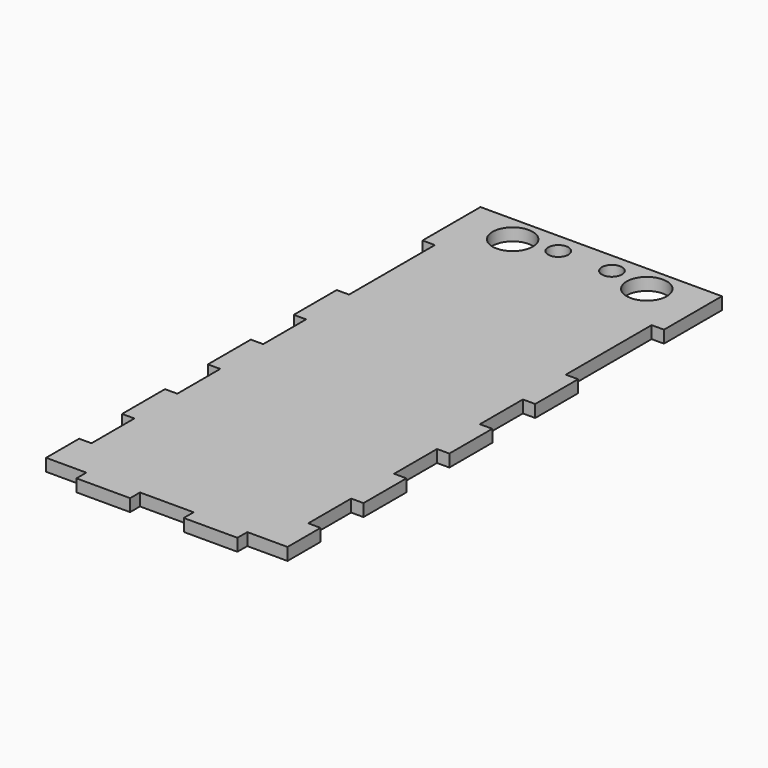
from build123d import *

# Parameters (mm, degrees)
F0_W     = 114.3
F0_H     = 262.89
F1_DEPTH = 5.842
F2_W     = 25.4
F2_H     = 5.842
F2_W_2   = 19.05
F2_W_3   = 5.842
F2_H_2   = 25.4
F3_DEPTH = 5.842
F4_R     = 4.7625
F4_R_2   = 9.525
F5_DEPTH = 5.842


# Not quite as in the source:
# - a feature names something its author has since deleted; it is built from what else it names


with BuildPart() as f1:
    # F0 (on Top) → F1 (new body)
    with BuildSketch(Plane.XY):
        with Locations((-21.309719372, 12.5171500933)):
            Rectangle(F0_W, F0_H)
    extrude(amount=-F1_DEPTH)

    # F2 (on face) → F3 (cut, through all)
    with BuildSketch(Plane.XY):
        with Locations((-21.309719372, -116.0068499067)):
            Rectangle(F2_W, F2_H)
        with Locations((-68.934719372, -116.0068499067)):
            Rectangle(F2_W_2, F2_H)
        with Locations((26.315280628, -116.0068499067)):
            Rectangle(F2_W_2, F2_H)
        with Locations((-75.538719372, -80.8278499067)):
            Rectangle(F2_W_3, F2_H_2)
        with Locations((32.919280628, -80.8278499067)):
            Rectangle(F2_W_3, F2_H_2)
        with Locations((32.919280628, -30.0278499067)):
            Rectangle(F2_W_3, F2_H_2)
        with Locations((-75.538719372, -30.0278499067)):
            Rectangle(F2_W_3, F2_H_2)
        with Locations((-75.538719372, 20.7721500933)):
            Rectangle(F2_W_3, F2_H_2)
        with Locations((32.919280628, 20.7721500933)):
            Rectangle(F2_W_3, F2_H_2)
        with Locations((-75.538719372, 71.5721500933)):
            Rectangle(F2_W_3, F2_H_2)
        with Locations((32.919280628, 71.5721500933)):
            Rectangle(F2_W_3, F2_H_2)
        with Locations((-75.538719372, 96.9721500933)):
            Rectangle(F2_W_3, F2_H_2)
        with Locations((32.919280628, 96.9721500933)):
            Rectangle(F2_W_3, F2_H_2)
    extrude(amount=-F3_DEPTH, mode=Mode.SUBTRACT)

    # F4 (on face) → F5 (cut, through all)
    with BuildSketch(Plane.XY):
        with Locations((-34.009719372, 134.4371500933)):
            Circle(F4_R)
        with Locations((-8.609719372, 134.4371500933)):
            Circle(F4_R)
        with Locations((-53.059719372, 131.2621500933)):
            Circle(F4_R_2)
        with Locations((10.440280628, 131.2621500933)):
            Circle(F4_R_2)
    extrude(amount=-F5_DEPTH, mode=Mode.SUBTRACT)


solid = f1.part
